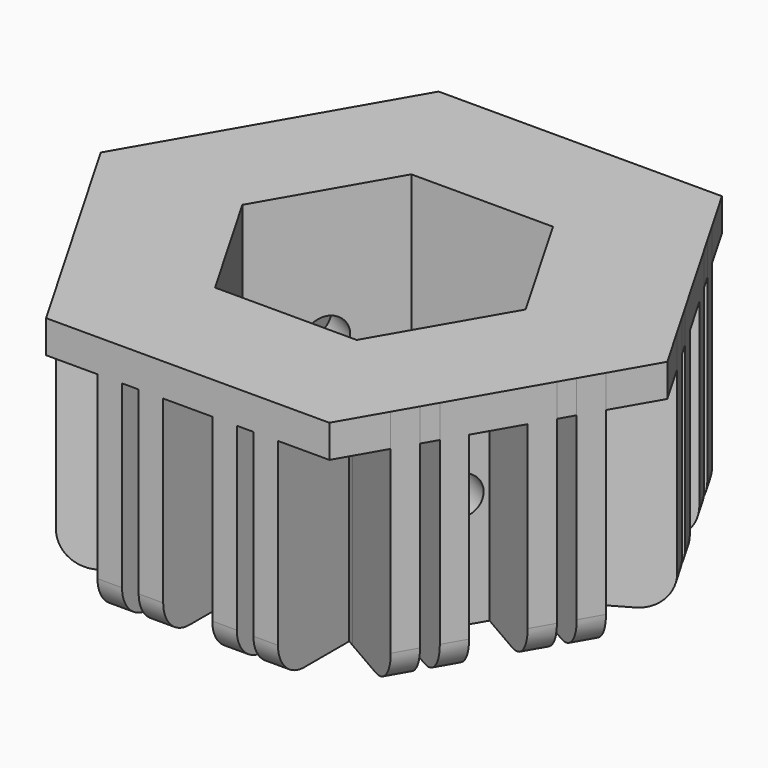
from build123d import *

# Parameters (mm, degrees)
F0_W            = 7.5
F0_H            = 25
F0_W_2          = 5.08
F0_W_3          = 15
F0_H_2          = 12.5
F1_DEPTH        = 75
F2_DEPTH        = 65
F3_R            = 10
F5_DEPTH        = 60
F6_R            = 6
F7_DEPTH        = 25
F7_COPIES_COUNT = 6


# Not quite as in the source:
# - a pattern or mirror of a feature is missing from the dataset's text; its kind, count and spacing are read off the source's solid


with BuildPart() as f1:
    # F0 (on Top) → F1 (new body)
    with BuildSketch(Plane.XY):
        with Locations((-23.83, 62.5)):
            Rectangle(F0_W, F0_H)
        with Locations((-17.54, 62.5)):
            Rectangle(F0_W_2, F0_H)
        with Locations((-11.25, 62.5)):
            Rectangle(F0_W, F0_H)
        with Locations((0, 62.5)):
            Rectangle(F0_W_3, F0_H)
        with Locations((11.25, 62.5)):
            Rectangle(F0_W, F0_H)
        with Locations((17.54, 62.5)):
            Rectangle(F0_W_2, F0_H)
        with Locations((23.83, 62.5)):
            Rectangle(F0_W, F0_H)
        Polygon((29.5112701892, 48.8849806364), (51.1619052838, 61.3849806364), (43.3012701892, 75), (27.58, 75), (27.58, 50), (27.58, 47.7699612727), align=None)
        Polygon((33.2612701892, 42.389790108), (54.9119052838, 54.889790108), (51.1619052838, 61.3849806364), (29.5112701892, 48.8849806364), align=None)
        Polygon((-27.58, 47.7699612727), (-20.08, 43.4398342538), (-20.08, 50), (-27.58, 50), align=None)
        Polygon((-27.58, 39.1097072349), (-22.4359526419, 36.139790108), (-21.6506350946, 37.5), (-20.08, 37.5), (-20.08, 43.4398342538), (-27.58, 47.7699612727), align=None)
        Polygon((-20.08, 37.5), (-15, 37.5), (-15, 50), (-20.08, 50), (-20.08, 43.4398342538), align=None)
        with Locations((-11.25, 43.75)):
            Rectangle(F0_W, F0_H_2)
        with Locations((0, 43.75)):
            Rectangle(F0_W_3, F0_H_2)
        with Locations((11.25, 43.75)):
            Rectangle(F0_W, F0_H_2)
        Polygon((15, 37.5), (20.08, 37.5), (20.08, 43.4398342538), (20.08, 50), (15, 50), align=None)
        Polygon((21.6506350946, 37.5), (22.4359526419, 36.139790108), (27.58, 39.1097072349), (27.58, 47.7699612727), (20.08, 43.4398342538), (20.08, 37.5), align=None)
        Polygon((20.08, 43.4398342538), (27.58, 47.7699612727), (27.58, 50), (20.08, 50), align=None)
        Polygon((27.58, 39.1097072349), (33.2612701892, 42.389790108), (29.5112701892, 48.8849806364), (27.58, 47.7699612727), align=None)
        Polygon((22.4359526419, 36.139790108), (24.9759526419, 31.7403810568), (35.8012701892, 37.9903810568), (33.2612701892, 42.389790108), (27.58, 39.1097072349), align=None)
        Polygon((35.8012701892, 37.9903810568), (57.4519052838, 50.4903810568), (54.9119052838, 54.889790108), (33.2612701892, 42.389790108), align=None)
        Polygon((24.9759526419, 31.7403810568), (28.7259526419, 25.2451905284), (39.5512701892, 31.4951905284), (35.8012701892, 37.9903810568), align=None)
        Polygon((39.5512701892, 31.4951905284), (61.2019052838, 43.9951905284), (57.4519052838, 50.4903810568), (35.8012701892, 37.9903810568), align=None)
        Polygon((28.7259526419, 25.2451905284), (36.2259526419, 12.2548094716), (47.0512701892, 18.5048094716), (39.5512701892, 31.4951905284), align=None)
        Polygon((47.0512701892, 18.5048094716), (68.7019052838, 31.0048094716), (61.2019052838, 43.9951905284), (39.5512701892, 31.4951905284), align=None)
        Polygon((36.2259526419, 12.2548094716), (39.9759526419, 5.7596189432), (50.8012701892, 12.0096189432), (47.0512701892, 18.5048094716), align=None)
        Polygon((50.8012701892, 12.0096189432), (72.4519052838, 24.5096189432), (68.7019052838, 31.0048094716), (47.0512701892, 18.5048094716), align=None)
        Polygon((42.5159526419, 1.360209892), (47.66, 4.3301270189), (53.3412701892, 7.610209892), (50.8012701892, 12.0096189432), (39.9759526419, 5.7596189432), align=None)
        Polygon((42.5159526419, -1.360209892), (47.66, -4.3301270189), (55.16, 0), (47.66, 4.3301270189), (42.5159526419, 1.360209892), (43.3012701892, 0), align=None)
        Polygon((47.66, 4.3301270189), (55.16, 0), (57.0912701892, 1.1150193636), (53.3412701892, 7.610209892), align=None)
        Polygon((53.3412701892, 7.610209892), (74.9919052838, 20.110209892), (72.4519052838, 24.5096189432), (50.8012701892, 12.0096189432), align=None)
        Polygon((57.0912701892, 1.1150193636), (78.7419052838, 13.6150193636), (74.9919052838, 20.110209892), (53.3412701892, 7.610209892), align=None)
        Polygon((57.0912701892, -1.1150193636), (78.7419052838, -13.6150193636), (86.6025403784, 0), (78.7419052838, 13.6150193636), (57.0912701892, 1.1150193636), (55.16, 0), align=None)
        Polygon((53.3412701892, -7.610209892), (74.9919052838, -20.110209892), (78.7419052838, -13.6150193636), (57.0912701892, -1.1150193636), align=None)
        Polygon((47.66, -4.3301270189), (53.3412701892, -7.610209892), (57.0912701892, -1.1150193636), (55.16, 0), align=None)
        Polygon((39.9759526419, -5.7596189432), (50.8012701892, -12.0096189432), (53.3412701892, -7.610209892), (47.66, -4.3301270189), (42.5159526419, -1.360209892), align=None)
        Polygon((50.8012701892, -12.0096189432), (72.4519052838, -24.5096189432), (74.9919052838, -20.110209892), (53.3412701892, -7.610209892), align=None)
        Polygon((47.0512701892, -18.5048094716), (68.7019052838, -31.0048094716), (72.4519052838, -24.5096189432), (50.8012701892, -12.0096189432), align=None)
        Polygon((36.2259526419, -12.2548094716), (47.0512701892, -18.5048094716), (50.8012701892, -12.0096189432), (39.9759526419, -5.7596189432), align=None)
        Polygon((28.7259526419, -25.2451905284), (39.5512701892, -31.4951905284), (47.0512701892, -18.5048094716), (36.2259526419, -12.2548094716), align=None)
        Polygon((39.5512701892, -31.4951905284), (61.2019052838, -43.9951905284), (68.7019052838, -31.0048094716), (47.0512701892, -18.5048094716), align=None)
        Polygon((24.9759526419, -31.7403810568), (35.8012701892, -37.9903810568), (39.5512701892, -31.4951905284), (28.7259526419, -25.2451905284), align=None)
        Polygon((35.8012701892, -37.9903810568), (57.4519052838, -50.4903810568), (61.2019052838, -43.9951905284), (39.5512701892, -31.4951905284), align=None)
        Polygon((27.58, -39.1097072349), (33.2612701892, -42.389790108), (35.8012701892, -37.9903810568), (24.9759526419, -31.7403810568), (22.4359526419, -36.139790108), align=None)
        Polygon((33.2612701892, -42.389790108), (54.9119052838, -54.889790108), (57.4519052838, -50.4903810568), (35.8012701892, -37.9903810568), align=None)
        Polygon((29.5112701892, -48.8849806364), (51.1619052838, -61.3849806364), (54.9119052838, -54.889790108), (33.2612701892, -42.389790108), align=None)
        Polygon((20.08, -43.4398342538), (27.58, -47.7699612727), (27.58, -39.1097072349), (22.4359526419, -36.139790108), (21.6506350946, -37.5), (20.08, -37.5), align=None)
        Polygon((27.58, -47.7699612727), (29.5112701892, -48.8849806364), (33.2612701892, -42.389790108), (27.58, -39.1097072349), align=None)
        Polygon((27.58, -75), (43.3012701892, -75), (51.1619052838, -61.3849806364), (29.5112701892, -48.8849806364), (27.58, -47.7699612727), (27.58, -50), align=None)
        with Locations((23.83, -62.5)):
            Rectangle(F0_W, F0_H)
        Polygon((20.08, -50), (27.58, -50), (27.58, -47.7699612727), (20.08, -43.4398342538), align=None)
        Polygon((15, -50), (20.08, -50), (20.08, -43.4398342538), (20.08, -37.5), (15, -37.5), align=None)
        with Locations((17.54, -62.5)):
            Rectangle(F0_W_2, F0_H)
        with Locations((11.25, -62.5)):
            Rectangle(F0_W, F0_H)
        with Locations((11.25, -43.75)):
            Rectangle(F0_W, F0_H_2)
        with Locations((0, -43.75)):
            Rectangle(F0_W_3, F0_H_2)
        with Locations((0, -62.5)):
            Rectangle(F0_W_3, F0_H)
        with Locations((-11.25, -62.5)):
            Rectangle(F0_W, F0_H)
        with Locations((-11.25, -43.75)):
            Rectangle(F0_W, F0_H_2)
        with Locations((-17.54, -62.5)):
            Rectangle(F0_W_2, F0_H)
        Polygon((-20.08, -50), (-15, -50), (-15, -37.5), (-20.08, -37.5), (-20.08, -43.4398342538), align=None)
        Polygon((-27.58, -47.7699612727), (-20.08, -43.4398342538), (-20.08, -37.5), (-21.6506350946, -37.5), (-22.4359526419, -36.139790108), (-27.58, -39.1097072349), align=None)
        Polygon((-27.58, -50), (-20.08, -50), (-20.08, -43.4398342538), (-27.58, -47.7699612727), align=None)
        with Locations((-23.83, -62.5)):
            Rectangle(F0_W, F0_H)
        Polygon((-43.3012701892, -75), (-27.58, -75), (-27.58, -50), (-27.58, -47.7699612727), (-29.5112701892, -48.8849806364), (-51.1619052838, -61.3849806364), align=None)
        Polygon((-29.5112701892, -48.8849806364), (-27.58, -47.7699612727), (-27.58, -39.1097072349), (-33.2612701892, -42.389790108), align=None)
        Polygon((-33.2612701892, -42.389790108), (-27.58, -39.1097072349), (-22.4359526419, -36.139790108), (-24.9759526419, -31.7403810568), (-35.8012701892, -37.9903810568), align=None)
        Polygon((-54.9119052838, -54.889790108), (-51.1619052838, -61.3849806364), (-29.5112701892, -48.8849806364), (-33.2612701892, -42.389790108), align=None)
        Polygon((-57.4519052838, -50.4903810568), (-54.9119052838, -54.889790108), (-33.2612701892, -42.389790108), (-35.8012701892, -37.9903810568), align=None)
        Polygon((-61.2019052838, -43.9951905284), (-57.4519052838, -50.4903810568), (-35.8012701892, -37.9903810568), (-39.5512701892, -31.4951905284), align=None)
        Polygon((-35.8012701892, -37.9903810568), (-24.9759526419, -31.7403810568), (-28.7259526419, -25.2451905284), (-39.5512701892, -31.4951905284), align=None)
        Polygon((-68.7019052838, -31.0048094716), (-61.2019052838, -43.9951905284), (-39.5512701892, -31.4951905284), (-47.0512701892, -18.5048094716), align=None)
        Polygon((-39.5512701892, -31.4951905284), (-28.7259526419, -25.2451905284), (-36.2259526419, -12.2548094716), (-47.0512701892, -18.5048094716), align=None)
        Polygon((-72.4519052838, -24.5096189432), (-68.7019052838, -31.0048094716), (-47.0512701892, -18.5048094716), (-50.8012701892, -12.0096189432), align=None)
        Polygon((-74.9919052838, -20.110209892), (-72.4519052838, -24.5096189432), (-50.8012701892, -12.0096189432), (-53.3412701892, -7.610209892), align=None)
        Polygon((-50.8012701892, -12.0096189432), (-39.9759526419, -5.7596189432), (-42.5159526419, -1.360209892), (-47.66, -4.3301270189), (-53.3412701892, -7.610209892), align=None)
        Polygon((-47.0512701892, -18.5048094716), (-36.2259526419, -12.2548094716), (-39.9759526419, -5.7596189432), (-50.8012701892, -12.0096189432), align=None)
        Polygon((-78.7419052838, -13.6150193636), (-74.9919052838, -20.110209892), (-53.3412701892, -7.610209892), (-57.0912701892, -1.1150193636), align=None)
        Polygon((-47.66, -4.3301270189), (-42.5159526419, -1.360209892), (-43.3012701892, 0), (-42.5159526419, 1.360209892), (-47.66, 4.3301270189), (-55.16, 0), align=None)
        Polygon((-57.0912701892, -1.1150193636), (-53.3412701892, -7.610209892), (-47.66, -4.3301270189), (-55.16, 0), align=None)
        Polygon((-86.6025403784, 0), (-78.7419052838, -13.6150193636), (-57.0912701892, -1.1150193636), (-55.16, 0), (-57.0912701892, 1.1150193636), (-78.7419052838, 13.6150193636), align=None)
        Polygon((-57.0912701892, 1.1150193636), (-55.16, 0), (-47.66, 4.3301270189), (-53.3412701892, 7.610209892), align=None)
        Polygon((-47.66, 4.3301270189), (-42.5159526419, 1.360209892), (-39.9759526419, 5.7596189432), (-50.8012701892, 12.0096189432), (-53.3412701892, 7.610209892), align=None)
        Polygon((-74.9919052838, 20.110209892), (-78.7419052838, 13.6150193636), (-57.0912701892, 1.1150193636), (-53.3412701892, 7.610209892), align=None)
        Polygon((-72.4519052838, 24.5096189432), (-74.9919052838, 20.110209892), (-53.3412701892, 7.610209892), (-50.8012701892, 12.0096189432), align=None)
        Polygon((-72.4519052838, 24.5096189432), (-50.8012701892, 12.0096189432), (-47.0512701892, 18.5048094716), (-68.7019052838, 31.0048094716), align=None)
        Polygon((-50.8012701892, 12.0096189432), (-39.9759526419, 5.7596189432), (-36.2259526419, 12.2548094716), (-47.0512701892, 18.5048094716), align=None)
        Polygon((-68.7019052838, 31.0048094716), (-47.0512701892, 18.5048094716), (-39.5512701892, 31.4951905284), (-61.2019052838, 43.9951905284), align=None)
        Polygon((-47.0512701892, 18.5048094716), (-36.2259526419, 12.2548094716), (-28.7259526419, 25.2451905284), (-39.5512701892, 31.4951905284), align=None)
        Polygon((-61.2019052838, 43.9951905284), (-39.5512701892, 31.4951905284), (-35.8012701892, 37.9903810568), (-57.4519052838, 50.4903810568), align=None)
        Polygon((-39.5512701892, 31.4951905284), (-28.7259526419, 25.2451905284), (-24.9759526419, 31.7403810568), (-35.8012701892, 37.9903810568), align=None)
        Polygon((-57.4519052838, 50.4903810568), (-35.8012701892, 37.9903810568), (-33.2612701892, 42.389790108), (-54.9119052838, 54.889790108), align=None)
        Polygon((-54.9119052838, 54.889790108), (-33.2612701892, 42.389790108), (-29.5112701892, 48.8849806364), (-51.1619052838, 61.3849806364), align=None)
        Polygon((-33.2612701892, 42.389790108), (-27.58, 39.1097072349), (-27.58, 47.7699612727), (-29.5112701892, 48.8849806364), align=None)
        Polygon((-35.8012701892, 37.9903810568), (-24.9759526419, 31.7403810568), (-22.4359526419, 36.139790108), (-27.58, 39.1097072349), (-33.2612701892, 42.389790108), align=None)
        Polygon((-29.5112701892, 48.8849806364), (-27.58, 47.7699612727), (-27.58, 50), (-27.58, 75), (-43.3012701892, 75), (-51.1619052838, 61.3849806364), align=None)
        Polygon((7.5, -37.5), (15, -37.5), (20.08, -37.5), (21.6506350946, -37.5), (22.4359526419, -36.139790108), (24.9759526419, -31.7403810568), (28.7259526419, -25.2451905284), (36.2259526419, -12.2548094716), (39.9759526419, -5.7596189432), (42.5159526419, -1.360209892), (43.3012701892, 0), (42.5159526419, 1.360209892), (39.9759526419, 5.7596189432), (36.2259526419, 12.2548094716), (28.7259526419, 25.2451905284), (24.9759526419, 31.7403810568), (22.4359526419, 36.139790108), (21.6506350946, 37.5), (20.08, 37.5), (15, 37.5), (7.5, 37.5), (-7.5, 37.5), (-15, 37.5), (-20.08, 37.5), (-21.6506350946, 37.5), (-22.4359526419, 36.139790108), (-24.9759526419, 31.7403810568), (-28.7259526419, 25.2451905284), (-36.2259526419, 12.2548094716), (-39.9759526419, 5.7596189432), (-42.5159526419, 1.360209892), (-43.3012701892, 0), (-42.5159526419, -1.360209892), (-39.9759526419, -5.7596189432), (-36.2259526419, -12.2548094716), (-28.7259526419, -25.2451905284), (-24.9759526419, -31.7403810568), (-22.4359526419, -36.139790108), (-21.6506350946, -37.5), (-20.08, -37.5), (-15, -37.5), (-7.5, -37.5), align=None)
    extrude(amount=F1_DEPTH)

    # F0 (on Top) → F2 (cut)
    with BuildSketch(Plane.XY):
        Polygon((27.58, -75), (43.3012701892, -75), (51.1619052838, -61.3849806364), (29.5112701892, -48.8849806364), (27.58, -47.7699612727), (27.58, -50), align=None)
        Polygon((33.2612701892, -42.389790108), (54.9119052838, -54.889790108), (57.4519052838, -50.4903810568), (35.8012701892, -37.9903810568), align=None)
        Polygon((39.5512701892, -31.4951905284), (61.2019052838, -43.9951905284), (68.7019052838, -31.0048094716), (47.0512701892, -18.5048094716), align=None)
        Polygon((50.8012701892, -12.0096189432), (72.4519052838, -24.5096189432), (74.9919052838, -20.110209892), (53.3412701892, -7.610209892), align=None)
        Polygon((57.0912701892, -1.1150193636), (78.7419052838, -13.6150193636), (86.6025403784, 0), (78.7419052838, 13.6150193636), (57.0912701892, 1.1150193636), (55.16, 0), align=None)
        Polygon((53.3412701892, 7.610209892), (74.9919052838, 20.110209892), (72.4519052838, 24.5096189432), (50.8012701892, 12.0096189432), align=None)
        Polygon((47.0512701892, 18.5048094716), (68.7019052838, 31.0048094716), (61.2019052838, 43.9951905284), (39.5512701892, 31.4951905284), align=None)
        Polygon((35.8012701892, 37.9903810568), (57.4519052838, 50.4903810568), (54.9119052838, 54.889790108), (33.2612701892, 42.389790108), align=None)
        Polygon((29.5112701892, 48.8849806364), (51.1619052838, 61.3849806364), (43.3012701892, 75), (27.58, 75), (27.58, 50), (27.58, 47.7699612727), align=None)
        with Locations((17.54, 62.5)):
            Rectangle(F0_W_2, F0_H)
        with Locations((0, 62.5)):
            Rectangle(F0_W_3, F0_H)
        with Locations((-17.54, 62.5)):
            Rectangle(F0_W_2, F0_H)
        Polygon((-29.5112701892, 48.8849806364), (-27.58, 47.7699612727), (-27.58, 50), (-27.58, 75), (-43.3012701892, 75), (-51.1619052838, 61.3849806364), align=None)
        Polygon((-57.4519052838, 50.4903810568), (-35.8012701892, 37.9903810568), (-33.2612701892, 42.389790108), (-54.9119052838, 54.889790108), align=None)
        Polygon((-68.7019052838, 31.0048094716), (-47.0512701892, 18.5048094716), (-39.5512701892, 31.4951905284), (-61.2019052838, 43.9951905284), align=None)
        Polygon((-72.4519052838, 24.5096189432), (-74.9919052838, 20.110209892), (-53.3412701892, 7.610209892), (-50.8012701892, 12.0096189432), align=None)
        Polygon((-86.6025403784, 0), (-78.7419052838, -13.6150193636), (-57.0912701892, -1.1150193636), (-55.16, 0), (-57.0912701892, 1.1150193636), (-78.7419052838, 13.6150193636), align=None)
        Polygon((-74.9919052838, -20.110209892), (-72.4519052838, -24.5096189432), (-50.8012701892, -12.0096189432), (-53.3412701892, -7.610209892), align=None)
        Polygon((-68.7019052838, -31.0048094716), (-61.2019052838, -43.9951905284), (-39.5512701892, -31.4951905284), (-47.0512701892, -18.5048094716), align=None)
        Polygon((-57.4519052838, -50.4903810568), (-54.9119052838, -54.889790108), (-33.2612701892, -42.389790108), (-35.8012701892, -37.9903810568), align=None)
        Polygon((-43.3012701892, -75), (-27.58, -75), (-27.58, -50), (-27.58, -47.7699612727), (-29.5112701892, -48.8849806364), (-51.1619052838, -61.3849806364), align=None)
        with Locations((-17.54, -62.5)):
            Rectangle(F0_W_2, F0_H)
        with Locations((0, -62.5)):
            Rectangle(F0_W_3, F0_H)
        with Locations((17.54, -62.5)):
            Rectangle(F0_W_2, F0_H)
    extrude(amount=F2_DEPTH, mode=Mode.SUBTRACT)

    # F3
    f3_edges = [f1.edges().sort_by_distance(p)[0] for p in [
        (76.866905, 16.862615, 0),
        (70.576905, 27.757214, 0),
        (59.326905, 47.242786, 0),
        (53.036905, 58.137385, 0),
        (23.83, 75, 0),
        (11.25, 75, 0),
        (-11.25, 75, 0),
        (-23.83, 75, 0),
        (-53.036905, 58.137385, 0),
        (-59.326905, 47.242786, 0),
        (-70.576905, 27.757214, 0),
        (-76.866905, 16.862615, 0),
        (-76.866905, -16.862615, 0),
        (-70.576905, -27.757214, 0),
        (-59.326905, -47.242786, 0),
        (-53.036905, -58.137385, 0),
        (-23.83, -75, 0),
        (-11.25, -75, 0),
        (11.25, -75, 0),
        (23.83, -75, 0),
        (53.036905, -58.137385, 0),
        (59.326905, -47.242786, 0),
        (70.576905, -27.757214, 0),
        (76.866905, -16.862615, 0),
    ]]
    fillet(f3_edges, radius=F3_R)

    # F4 (on face) → F5 (cut)
    with BuildSketch(Plane.XY.offset(75)):
        Polygon((-21.6506350946, -37.5), (21.6506350946, -37.5), (43.3012701892, 0), (21.6506350946, 37.5), (-21.6506350946, 37.5), (-43.3012701892, 0), align=None)
    extrude(amount=-F5_DEPTH, mode=Mode.SUBTRACT)

    # F6 (on face) → F7 (cut)
    with BuildSketch(Plane.XZ.offset(-37.5)):
        with Locations((0, 35)):
            Circle(F6_R)
    f7 = extrude(amount=-F7_DEPTH, mode=Mode.SUBTRACT)

    # F7_copies: F7 ×6 about axis
    f7_copies_axis = Axis((0, 0, 0), (0, 0, 1))
    for i in range(1, F7_COPIES_COUNT):
        add(f7.rotate(f7_copies_axis, i * 360 / F7_COPIES_COUNT), mode=Mode.SUBTRACT)


solid = f1.part
